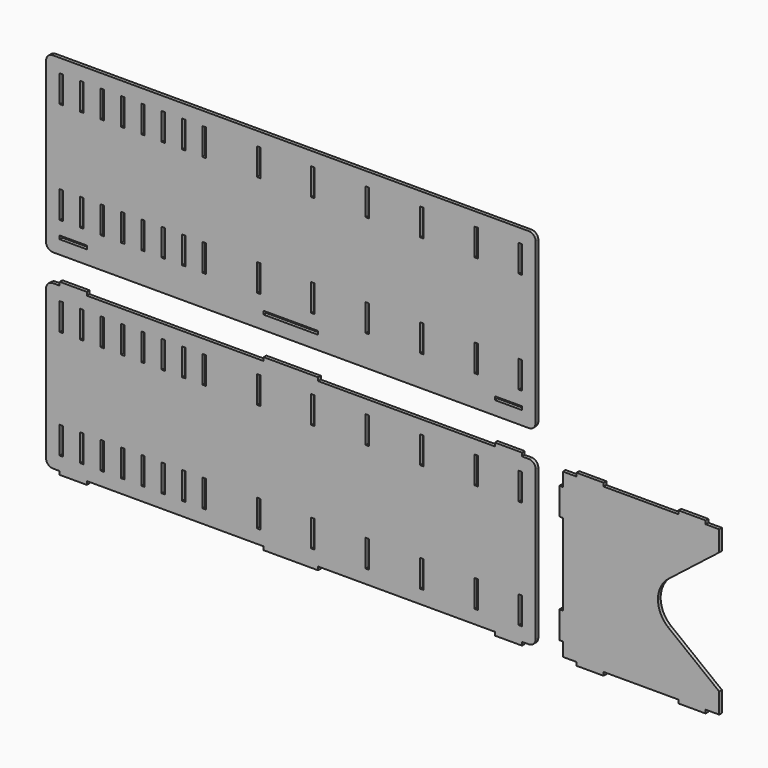
from build123d import *

# Parameters (mm, degrees)
F1_W     = 50.8
F1_H     = 6.35
F1_W_2   = 6.35
F1_H_2   = 50.8
F1_W_3   = 101.6
F2_DEPTH = 6.35


# Not quite as in the source:
# - a variable given as a bare number and used for a length is read in inches; the dataset says mm whatever the document's units were
# - a feature names something its author has since deleted; it is built from what else it names


with BuildPart() as f2:
    # F1 (on Front) → F2 (new body)
    with BuildSketch(Plane.XZ):
        with BuildLine():
            ThreePointArc((-457.2, 215.9), (-453.4802561211, 206.9197438789), (-444.5, 203.2))
            Line((-444.5, 203.2), (444.5, 203.2))
            ThreePointArc((444.5, 203.2), (453.4802561211, 206.9197438789), (457.2, 215.9))
            Line((457.2, 215.9), (457.2, 514.35))
            ThreePointArc((457.2, 514.35), (453.4802561211, 523.3302561211), (444.5, 527.05))
            Line((444.5, 527.05), (-444.5, 527.05))
            ThreePointArc((-444.5, 527.05), (-453.4802561211, 523.3302561211), (-457.2, 514.35))
            Line((-457.2, 514.35), (-457.2, 215.9))
        make_face()
        with Locations((-406.4, 231.775)):
            Rectangle(F1_W, F1_H, mode=Mode.SUBTRACT)
        with Locations((-428.625, 285.75)):
            Rectangle(F1_W_2, F1_H_2, mode=Mode.SUBTRACT)
        with Locations((-390.525, 285.75)):
            Rectangle(F1_W_2, F1_H_2, mode=Mode.SUBTRACT)
        with Locations((-352.425, 285.75)):
            Rectangle(F1_W_2, F1_H_2, mode=Mode.SUBTRACT)
        with Locations((-314.325, 285.75)):
            Rectangle(F1_W_2, F1_H_2, mode=Mode.SUBTRACT)
        with Locations((-276.225, 285.75)):
            Rectangle(F1_W_2, F1_H_2, mode=Mode.SUBTRACT)
        with Locations((-238.125, 285.75)):
            Rectangle(F1_W_2, F1_H_2, mode=Mode.SUBTRACT)
        with Locations((-200.025, 285.75)):
            Rectangle(F1_W_2, F1_H_2, mode=Mode.SUBTRACT)
        with Locations((-161.925, 285.75)):
            Rectangle(F1_W_2, F1_H_2, mode=Mode.SUBTRACT)
        with Locations((0, 231.775)):
            Rectangle(F1_W_3, F1_H, mode=Mode.SUBTRACT)
        with Locations((-60.325, 285.75)):
            Rectangle(F1_W_2, F1_H_2, mode=Mode.SUBTRACT)
        with Locations((41.275, 285.75)):
            Rectangle(F1_W_2, F1_H_2, mode=Mode.SUBTRACT)
        with Locations((142.875, 285.75)):
            Rectangle(F1_W_2, F1_H_2, mode=Mode.SUBTRACT)
        with Locations((-428.625, 476.25)):
            Rectangle(F1_W_2, F1_H_2, mode=Mode.SUBTRACT)
        with Locations((-390.525, 476.25)):
            Rectangle(F1_W_2, F1_H_2, mode=Mode.SUBTRACT)
        with Locations((-352.425, 476.25)):
            Rectangle(F1_W_2, F1_H_2, mode=Mode.SUBTRACT)
        with Locations((-314.325, 476.25)):
            Rectangle(F1_W_2, F1_H_2, mode=Mode.SUBTRACT)
        with Locations((-276.225, 476.25)):
            Rectangle(F1_W_2, F1_H_2, mode=Mode.SUBTRACT)
        with Locations((-238.125, 476.25)):
            Rectangle(F1_W_2, F1_H_2, mode=Mode.SUBTRACT)
        with Locations((-200.025, 476.25)):
            Rectangle(F1_W_2, F1_H_2, mode=Mode.SUBTRACT)
        with Locations((-161.925, 476.25)):
            Rectangle(F1_W_2, F1_H_2, mode=Mode.SUBTRACT)
        with Locations((-60.325, 476.25)):
            Rectangle(F1_W_2, F1_H_2, mode=Mode.SUBTRACT)
        with Locations((41.275, 476.25)):
            Rectangle(F1_W_2, F1_H_2, mode=Mode.SUBTRACT)
        with Locations((142.875, 476.25)):
            Rectangle(F1_W_2, F1_H_2, mode=Mode.SUBTRACT)
        with Locations((406.4, 231.775)):
            Rectangle(F1_W, F1_H, mode=Mode.SUBTRACT)
        with Locations((244.475, 285.75)):
            Rectangle(F1_W_2, F1_H_2, mode=Mode.SUBTRACT)
        with Locations((346.075, 285.75)):
            Rectangle(F1_W_2, F1_H_2, mode=Mode.SUBTRACT)
        with Locations((428.625, 285.75)):
            Rectangle(F1_W_2, F1_H_2, mode=Mode.SUBTRACT)
        with Locations((244.475, 476.25)):
            Rectangle(F1_W_2, F1_H_2, mode=Mode.SUBTRACT)
        with Locations((346.075, 476.25)):
            Rectangle(F1_W_2, F1_H_2, mode=Mode.SUBTRACT)
        with Locations((428.625, 476.25)):
            Rectangle(F1_W_2, F1_H_2, mode=Mode.SUBTRACT)
    extrude(amount=F2_DEPTH)


with BuildPart() as f2b:
    # F1 (on Front) → F2, piece 2 (new body)
    with BuildSketch(Plane.XZ):
        with BuildLine():
            Line((-431.8, 152.4), (-444.5, 152.4))
            ThreePointArc((-444.5, 152.4), (-453.4802561211, 148.6802561211), (-457.2, 139.7))
            Line((-457.2, 139.7), (-457.2, -139.7))
            ThreePointArc((-457.2, -139.7), (-453.4802561211, -148.6802561211), (-444.5, -152.4))
            Line((-444.5, -152.4), (-431.8, -152.4))
            Line((-431.8, -152.4), (-431.8, -158.75))
            Line((-431.8, -158.75), (-381, -158.75))
            Line((-381, -158.75), (-381, -152.4))
            Line((-381, -152.4), (-50.8, -152.4))
            Line((-50.8, -152.4), (-50.8, -158.75))
            Line((-50.8, -158.75), (50.8, -158.75))
            Line((50.8, -158.75), (50.8, -152.4))
            Line((50.8, -152.4), (381, -152.4))
            Line((381, -152.4), (381, -158.75))
            Line((381, -158.75), (431.8, -158.75))
            Line((431.8, -158.75), (431.8, -152.4))
            Line((431.8, -152.4), (444.5, -152.4))
            ThreePointArc((444.5, -152.4), (453.4802561211, -148.6802561211), (457.2, -139.7))
            Line((457.2, -139.7), (457.2, 139.7))
            ThreePointArc((457.2, 139.7), (453.4802561211, 148.6802561211), (444.5, 152.4))
            Line((444.5, 152.4), (431.8, 152.4))
            Line((431.8, 152.4), (431.8, 158.75))
            Line((431.8, 158.75), (381, 158.75))
            Line((381, 158.75), (381, 152.4))
            Line((381, 152.4), (50.8, 152.4))
            Line((50.8, 152.4), (50.8, 158.75))
            Line((50.8, 158.75), (-50.8, 158.75))
            Line((-50.8, 158.75), (-50.8, 152.4))
            Line((-50.8, 152.4), (-381, 152.4))
            Line((-381, 152.4), (-381, 158.75))
            Line((-381, 158.75), (-431.8, 158.75))
            Line((-431.8, 158.75), (-431.8, 152.4))
        make_face()
        with Locations((-428.625, -101.6)):
            Rectangle(F1_W_2, F1_H_2, mode=Mode.SUBTRACT)
        with Locations((-390.525, -101.6)):
            Rectangle(F1_W_2, F1_H_2, mode=Mode.SUBTRACT)
        with Locations((-352.425, -101.6)):
            Rectangle(F1_W_2, F1_H_2, mode=Mode.SUBTRACT)
        with Locations((-314.325, -101.6)):
            Rectangle(F1_W_2, F1_H_2, mode=Mode.SUBTRACT)
        with Locations((-276.225, -101.6)):
            Rectangle(F1_W_2, F1_H_2, mode=Mode.SUBTRACT)
        with Locations((-238.125, -101.6)):
            Rectangle(F1_W_2, F1_H_2, mode=Mode.SUBTRACT)
        with Locations((-200.025, -101.6)):
            Rectangle(F1_W_2, F1_H_2, mode=Mode.SUBTRACT)
        with Locations((-161.925, -101.6)):
            Rectangle(F1_W_2, F1_H_2, mode=Mode.SUBTRACT)
        with Locations((-60.325, -101.6)):
            Rectangle(F1_W_2, F1_H_2, mode=Mode.SUBTRACT)
        with Locations((41.275, -101.6)):
            Rectangle(F1_W_2, F1_H_2, mode=Mode.SUBTRACT)
        with Locations((142.875, -101.6)):
            Rectangle(F1_W_2, F1_H_2, mode=Mode.SUBTRACT)
        with Locations((-428.625, 101.6)):
            Rectangle(F1_W_2, F1_H_2, mode=Mode.SUBTRACT)
        with Locations((-390.525, 101.6)):
            Rectangle(F1_W_2, F1_H_2, mode=Mode.SUBTRACT)
        with Locations((-352.425, 101.6)):
            Rectangle(F1_W_2, F1_H_2, mode=Mode.SUBTRACT)
        with Locations((-314.325, 101.6)):
            Rectangle(F1_W_2, F1_H_2, mode=Mode.SUBTRACT)
        with Locations((-276.225, 101.6)):
            Rectangle(F1_W_2, F1_H_2, mode=Mode.SUBTRACT)
        with Locations((-238.125, 101.6)):
            Rectangle(F1_W_2, F1_H_2, mode=Mode.SUBTRACT)
        with Locations((-200.025, 101.6)):
            Rectangle(F1_W_2, F1_H_2, mode=Mode.SUBTRACT)
        with Locations((-161.925, 101.6)):
            Rectangle(F1_W_2, F1_H_2, mode=Mode.SUBTRACT)
        with Locations((-60.325, 101.6)):
            Rectangle(F1_W_2, F1_H_2, mode=Mode.SUBTRACT)
        with Locations((41.275, 101.6)):
            Rectangle(F1_W_2, F1_H_2, mode=Mode.SUBTRACT)
        with Locations((142.875, 101.6)):
            Rectangle(F1_W_2, F1_H_2, mode=Mode.SUBTRACT)
        with Locations((244.475, -101.6)):
            Rectangle(F1_W_2, F1_H_2, mode=Mode.SUBTRACT)
        with Locations((346.075, -101.6)):
            Rectangle(F1_W_2, F1_H_2, mode=Mode.SUBTRACT)
        with Locations((428.625, -101.6)):
            Rectangle(F1_W_2, F1_H_2, mode=Mode.SUBTRACT)
        with Locations((244.475, 101.6)):
            Rectangle(F1_W_2, F1_H_2, mode=Mode.SUBTRACT)
        with Locations((346.075, 101.6)):
            Rectangle(F1_W_2, F1_H_2, mode=Mode.SUBTRACT)
        with Locations((428.625, 101.6)):
            Rectangle(F1_W_2, F1_H_2, mode=Mode.SUBTRACT)
    extrude(amount=F2_DEPTH)


with BuildPart() as f2c:
    # F1 (on Front) → F2, piece 3 (new body)
    with BuildSketch(Plane.XZ):
        with BuildLine():
            Line((533.4, 152.4), (508, 152.4))
            Line((508, 152.4), (508, 127))
            Line((508, 127), (501.65, 127))
            Line((501.65, 127), (501.65, 76.2))
            Line((501.65, 76.2), (508, 76.2))
            Line((508, 76.2), (508, -76.2))
            Line((508, -76.2), (508, -127))
            Line((508, -127), (508, -152.4))
            Line((508, -152.4), (533.4, -152.4))
            Line((533.4, -152.4), (533.4, -158.75))
            Line((533.4, -158.75), (584.2, -158.75))
            Line((584.2, -158.75), (584.2, -152.4))
            Line((584.2, -152.4), (723.9, -152.4))
            Line((723.9, -152.4), (723.9, -158.75))
            Line((723.9, -158.75), (774.7, -158.75))
            Line((774.7, -158.75), (774.7, -152.4))
            Line((774.7, -152.4), (800.1, -152.4))
            Line((800.1, -152.4), (800.1, -114.3))
            Line((800.1, -114.3), (705.167824621, -40.0052540512))
            ThreePointArc((705.167824621, -40.0052540512), (685.6762843132, 0), (705.167824621, 40.0052540512))
            Line((705.167824621, 40.0052540512), (800.1, 114.3))
            Line((800.1, 114.3), (800.1, 152.4))
            Line((800.1, 152.4), (774.7, 152.4))
            Line((774.7, 152.4), (774.7, 158.75))
            Line((774.7, 158.75), (723.9, 158.75))
            Line((723.9, 158.75), (723.9, 152.4))
            Line((723.9, 152.4), (584.2, 152.4))
            Line((584.2, 152.4), (584.2, 158.75))
            Line((584.2, 158.75), (533.4, 158.75))
            Line((533.4, 158.75), (533.4, 152.4))
        make_face()
        with Locations((504.825, -101.6)):
            Rectangle(F1_W_2, F1_H_2)
    extrude(amount=F2_DEPTH)


solid = Compound([f2.part, f2b.part, f2c.part])
